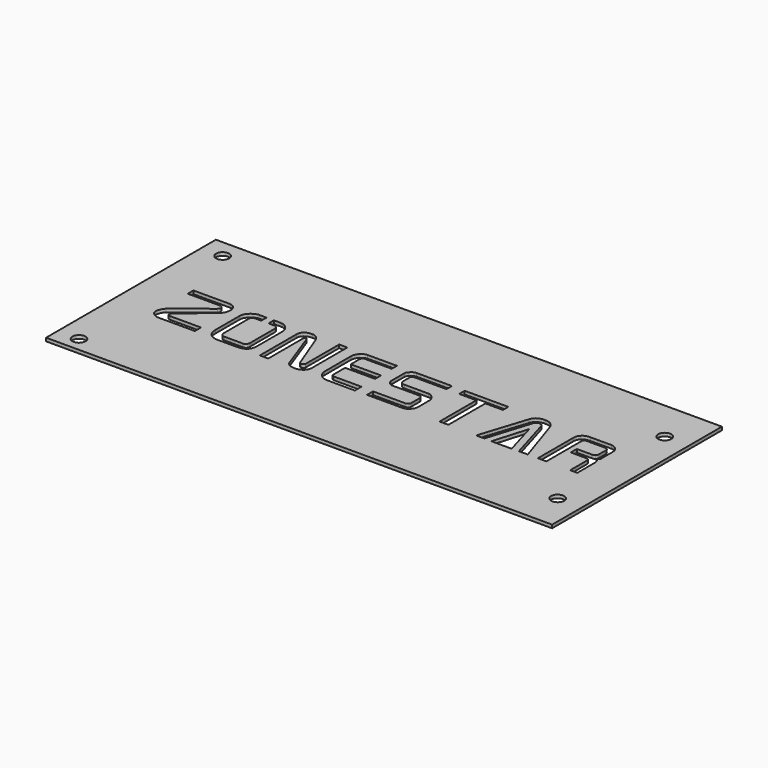
from build123d import *

# Parameters (mm, degrees)
F0_W     = 155
F0_H     = 65
F0_R     = 2
F1_DEPTH = 1


# Not quite as in the source:
# - the dataset's text gives a spline's control points without its knots; the knots are read off the source's solid


with BuildPart() as f1:
    # F0 (on Top) → F1 (new body)
    with BuildSketch(Plane.XY):
        with Locations((0.0922121108, -0.4517037495)):
            Rectangle(F0_W, F0_H)
        with Locations((-70.8632841706, -28.5362548381)):
            Circle(F0_R, mode=Mode.SUBTRACT)
        with Locations((70.1367158294, -21.5362548381)):
            Circle(F0_R, mode=Mode.SUBTRACT)
        Polygon((45.469336, -8.307439), (39.270354, -8.307439), (42.393256, 2.334635), align=None, mode=Mode.SUBTRACT)
        with BuildLine():
            add(Edge.make_bspline(
                [(-54.423643, 5.266161), (-54.520325, 5.636939), (-54.790085, 6.060127), (-55.30921, 5.999047)],
                knots=[0, 0, 0, 0, 1, 1, 1, 1], degree=3))
            Line((-55.30921, 5.999047), (-65.172596, 5.999047))
            Line((-65.172596, 5.999047), (-65.172596, 8.167165))
            Line((-65.172596, 8.167165), (-54.026665, 8.167165))
            add(Edge.make_bspline(
                [(-54.026665, 8.167165), (-52.805193, 8.228245), (-51.793658, 6.852856), (-51.797479, 5.785286)],
                knots=[0, 0, 0, 0, 1, 1, 1, 1], degree=3))
            add(Edge.make_bspline(
                [(-51.797479, 5.785286), (-51.800629, 4.896518), (-52.07231, 3.892018), (-52.74412, 3.250733)],
                knots=[0, 0, 0, 0, 1, 1, 1, 1], degree=3))
            Line((-52.74412, 3.250733), (-61.294422, -4.139179))
            add(Edge.make_bspline(
                [(-61.294422, -4.139179), (-61.2949949402, -4.1395245064), (-61.2950082917, -4.1395281699), (-61.3406298874, -4.1671100697), (-62.1897265938, -4.692143), (-62.027305, -5.207952)],
                knots=[0, 0, 0, 0, 0.0208333333, 0.03125, 1, 1, 1, 1], degree=3))
            add(Edge.make_bspline(
                [(-62.027305, -5.207952), (-61.8797565625, -5.6765360625), (-61.2435394271, -5.6963794323), (-61.1740917839, -5.6965692578), (-61.1740246232, -5.6965409216), (-61.172275, -5.69654)],
                knots=[0, 0, 0, 0, 0.9375, 0.9583333333, 1, 1, 1, 1], degree=3))
            Line((-61.172275, -5.69654), (-51.766942, -5.69654))
            Line((-51.766942, -5.69654), (-51.766942, -8.047872))
            Line((-51.766942, -8.047872), (-62.973946, -8.047872))
            add(Edge.make_bspline(
                [(-62.973946, -8.047872), (-64.042733, -8.078322), (-65.507059, -6.99161), (-65.539036, -5.940845)],
                knots=[0, 0, 0, 0, 1, 1, 1, 1], degree=3))
            add(Edge.make_bspline(
                [(-65.539036, -5.940845), (-65.565623, -5.067222), (-64.989373, -3.83381), (-64.348102, -3.284142)],
                knots=[0, 0, 0, 0, 1, 1, 1, 1], degree=3))
            Line((-64.348102, -3.284142), (-54.790085, 4.319531))
            add(Edge.make_bspline(
                [(-54.790085, 4.319531), (-54.423643, 4.624895), (-54.338273, 4.938748), (-54.423643, 5.266161)],
                knots=[0, 0, 0, 0, 1, 1, 1, 1], degree=3))
        make_face(mode=Mode.SUBTRACT)
        with BuildLine():
            Line((-38.636265, 6.060218), (-40.482756, 6.059882))
            Line((-40.482756, 6.059882), (-40.482755, 8.106095))
            Line((-40.482755, 8.106095), (-38.345683, 8.10592))
            add(Edge.make_bspline(
                [(-35.246532, 4.981721), (-35.246532, 6.428433), (-36.834187, 8.10592), (-38.345683, 8.10592)],
                knots=[0, 0, 0, 0, 1, 1, 1, 1], degree=3))
            Line((-35.246532, 4.981721), (-35.246532, -4.812387))
            add(Edge.make_bspline(
                [(-38.701388, -8.200429), (-36.69326, -8.157304), (-35.268125, -7.360324), (-35.246532, -4.812387)],
                knots=[0, 0, 0, 0, 1, 1, 1, 1], degree=3))
            Line((-38.701388, -8.200429), (-44.697956, -8.200429))
            add(Edge.make_bspline(
                [(-48.316136, -4.465362), (-48.251358, -6.879897), (-46.814048, -8.200429), (-44.697956, -8.200429)],
                knots=[0, 0, 0, 0, 1, 1, 1, 1], degree=3))
            Line((-48.316136, -4.465362), (-48.302118, 4.692146))
            add(Edge.make_bspline(
                [(-45.033966, 8.10592), (-45.984047, 8.10592), (-48.345306, 6.873016), (-48.302118, 4.692146)],
                knots=[0, 0, 0, 0, 1, 1, 1, 1], degree=3))
            Line((-45.033966, 8.10592), (-42.724205, 8.10592))
            Line((-42.724205, 8.10592), (-42.744882, 6.059882))
            Line((-42.744882, 6.059882), (-44.712989, 6.060218))
            add(Edge.make_bspline(
                [(-45.690264, 5.082949), (-45.690264, 5.464662), (-45.323727, 6.060218), (-44.712989, 6.060218)],
                knots=[0, 0, 0, 0, 1, 1, 1, 1], degree=3))
            Line((-45.690264, 5.082949), (-45.690264, -4.50575))
            add(Edge.make_bspline(
                [(-44.438112, -5.910207), (-45.270239, -5.902257), (-45.629189, -5.368415), (-45.690264, -4.50575)],
                knots=[0, 0, 0, 0, 1, 1, 1, 1], degree=3))
            Line((-44.438112, -5.910207), (-38.727779, -5.910207))
            add(Edge.make_bspline(
                [(-37.597871, -4.597264), (-37.636046, -5.467557), (-37.941457, -5.910207), (-38.727779, -5.910207)],
                knots=[0, 0, 0, 0, 1, 1, 1, 1], degree=3))
            Line((-37.597871, -4.597264), (-37.597871, 4.930313))
            add(Edge.make_bspline(
                [(-38.636265, 6.060218), (-37.949187, 6.051991), (-37.605504, 5.487612), (-37.597871, 4.930313)],
                knots=[0, 0, 0, 0, 1, 1, 1, 1], degree=3))
        make_face(mode=Mode.SUBTRACT)
        with BuildLine():
            add(Edge.make_bspline(
                [(-28.782152, 5.759499), (-29.006319, 5.729049), (-29.165424, 5.484194), (-29.170821, 5.198091)],
                knots=[0, 0, 0, 0, 1, 1, 1, 1], degree=3))
            Line((-29.170821, 5.198091), (-29.170821, -8.211027))
            Line((-29.170821, -8.211027), (-31.74036, -8.211027))
            Line((-31.74036, -8.211027), (-31.74036, 5.910654))
            add(Edge.make_bspline(
                [(-31.74036, 5.910654), (-31.675598, 7.357366), (-30.714749, 8.210275), (-28.825337, 8.264266)],
                knots=[0, 0, 0, 0, 1, 1, 1, 1], degree=3))
            add(Edge.make_bspline(
                [(-28.825337, 8.264266), (-26.9949700938, 8.31657075), (-26.2305613594, 6.1368576556), (-26.1915039655, 6.0201141621), (-26.1915066754, 6.0200826051), (-26.191019, 6.018617)],
                knots=[0, 0, 0, 0, 0.96875, 0.9791666667, 1, 1, 1, 1], degree=3))
            Line((-26.191019, 6.018617), (-21.937244, -5.036892))
            add(Edge.make_bspline(
                [(-21.937244, -5.036892), (-21.834677, -5.263602), (-21.553159, -5.453479), (-21.089727, -5.366187)],
                knots=[0, 0, 0, 0, 1, 1, 1, 1], degree=3))
            add(Edge.make_bspline(
                [(-21.089727, -5.366187), (-20.671826, -5.28752), (-20.468935, -5.047684), (-20.468935, -4.712982)],
                knots=[0, 0, 0, 0, 1, 1, 1, 1], degree=3))
            Line((-20.468935, -4.712982), (-20.468935, 8.091524))
            Line((-20.468935, 8.091524), (-17.964172, 8.091524))
            Line((-17.964172, 8.091524), (-17.964172, -5.533519))
            add(Edge.make_bspline(
                [(-17.964172, -5.533519), (-17.942573, -7.174572), (-19.608218, -8.198607), (-20.911044, -8.198607)],
                knots=[0, 0, 0, 0, 1, 1, 1, 1], degree=3))
            add(Edge.make_bspline(
                [(-20.911044, -8.198607), (-22.213871, -8.198607), (-23.402846, -7.8026), (-23.858999, -6.742715)],
                knots=[0, 0, 0, 0, 1, 1, 1, 1], degree=3))
            Line((-23.858999, -6.742715), (-28.263925, 5.327641))
            add(Edge.make_bspline(
                [(-28.263925, 5.327641), (-28.39888, 5.640739), (-28.557983, 5.790003), (-28.782152, 5.759499)],
                knots=[0, 0, 0, 0, 1, 1, 1, 1], degree=3))
        make_face(mode=Mode.SUBTRACT)
        with BuildLine():
            Line((-2.784456, 6.083385), (-11.054481, 6.083385))
            add(Edge.make_bspline(
                [(-11.702271, 5.737913), (-11.544786, 5.939612), (-11.351384, 6.083385), (-11.054481, 6.083385)],
                knots=[0, 0, 0, 0, 1, 1, 1, 1], degree=3))
            add(Edge.make_bspline(
                [(-11.896604, 4.96057), (-11.891354, 5.268261), (-11.859779, 5.536203), (-11.702271, 5.737913)],
                knots=[0, 0, 0, 0, 1, 1, 1, 1], degree=3))
            Line((-11.896604, 4.96057), (-11.896604, 1.80802))
            Line((-11.896604, 1.80802), (-2.633301, 1.80802))
            Line((-2.633301, 1.80802), (-2.633301, -0.459213))
            Line((-2.633301, -0.459213), (-11.810234, -0.459213))
            Line((-11.810234, -0.459213), (-11.810234, -4.993707))
            add(Edge.make_bspline(
                [(-11.540324, -5.506534), (-11.698656, -5.377504), (-11.815633, -5.242024), (-11.810234, -4.993707)],
                knots=[0, 0, 0, 0, 1, 1, 1, 1], degree=3))
            add(Edge.make_bspline(
                [(-10.881741, -5.663082), (-11.167851, -5.657832), (-11.381991, -5.635557), (-11.540324, -5.506534)],
                knots=[0, 0, 0, 0, 1, 1, 1, 1], degree=3))
            Line((-10.881741, -5.663082), (-2.633301, -5.663082))
            Line((-2.633301, -5.663082), (-2.633301, -8.189427))
            Line((-2.633301, -8.189427), (-11.227228, -8.189427))
            add(Edge.make_bspline(
                [(-13.451282, -7.239349), (-12.872516, -7.802097), (-11.993773, -8.162442), (-11.227228, -8.189427)],
                knots=[0, 0, 0, 0, 1, 1, 1, 1], degree=3))
            add(Edge.make_bspline(
                [(-14.466143, -5.036892), (-14.449951, -5.862807), (-14.030051, -6.676602), (-13.451282, -7.239349)],
                knots=[0, 0, 0, 0, 1, 1, 1, 1], degree=3))
            Line((-14.466143, -5.036892), (-14.466143, 5.176496))
            add(Edge.make_bspline(
                [(-13.616615, 7.184624), (-14.104807, 6.682724), (-14.468763, 5.882731), (-14.466143, 5.176496)],
                knots=[0, 0, 0, 0, 1, 1, 1, 1], degree=3))
            add(Edge.make_bspline(
                [(-11.745456, 8.091524), (-12.522793, 8.069983), (-13.128423, 7.686523), (-13.616615, 7.184624)],
                knots=[0, 0, 0, 0, 1, 1, 1, 1], degree=3))
            Line((-11.745456, 8.091524), (-2.784456, 8.091524))
            Line((-2.784456, 8.091524), (-2.784456, 6.083385))
        make_face(mode=Mode.SUBTRACT)
        with Locations((-70.8632841706, 26.4637451619)):
            Circle(F0_R, mode=Mode.SUBTRACT)
        with BuildLine():
            add(Edge.make_bspline(
                [(1.598881, 7.314182), (1.958971, 7.680189), (2.396462, 8.104167), (3.175141, 8.134707)],
                knots=[0, 0, 0, 0, 1, 1, 1, 1], degree=3))
            Line((3.175141, 8.134707), (14.036327, 8.134707))
            Line((14.036327, 8.134707), (14.036327, 6.040211))
            Line((14.036327, 6.040211), (4.125234, 6.040211))
            add(Edge.make_bspline(
                [(4.125234, 6.040211), (3.850397, 6.024941), (3.721074, 5.94307), (3.585414, 5.802682)],
                knots=[0, 0, 0, 0, 1, 1, 1, 1], degree=3))
            add(Edge.make_bspline(
                [(3.585414, 5.802682), (3.449762, 5.662334), (3.361854, 5.484259), (3.369482, 5.262861)],
                knots=[0, 0, 0, 0, 1, 1, 1, 1], degree=3))
            Line((3.369482, 5.262861), (3.369482, 2.563776))
            add(Edge.make_bspline(
                [(3.369482, 2.563776), (3.392357, 2.174428), (3.530417, 2.023619), (3.760562, 1.84596)],
                knots=[0, 0, 0, 0, 1, 1, 1, 1], degree=3))
            add(Edge.make_bspline(
                [(3.760562, 1.84596), (3.990684, 1.668301), (4.271777, 1.570501), (4.729839, 1.570501)],
                knots=[0, 0, 0, 0, 1, 1, 1, 1], degree=3))
            Line((4.729839, 1.570501), (12.092972, 1.570501))
            add(Edge.make_bspline(
                [(12.092972, 1.570501), (12.843482, 1.570501), (13.360134, 1.120618), (13.788002, 0.631214)],
                knots=[0, 0, 0, 0, 1, 1, 1, 1], degree=3))
            add(Edge.make_bspline(
                [(13.788002, 0.631214), (14.215869, 0.141821), (14.511354, -0.44272), (14.511354, -1.23656)],
                knots=[0, 0, 0, 0, 1, 1, 1, 1], degree=3))
            Line((14.511354, -1.23656), (14.511354, -5.036892))
            add(Edge.make_bspline(
                [(14.511354, -5.036892), (14.511354, -6.115047), (14.283234, -6.557255), (13.838267, -7.102385)],
                knots=[0, 0, 0, 0, 1, 1, 1, 1], degree=3))
            add(Edge.make_bspline(
                [(13.838267, -7.102385), (13.393307, -7.647522), (12.782012, -8.124657), (11.963402, -8.124657)],
                knots=[0, 0, 0, 0, 1, 1, 1, 1], degree=3))
            Line((11.963402, -8.124657), (1.037469, -8.124657))
            Line((1.037469, -8.124657), (1.037469, -5.814222))
            Line((1.037469, -5.814222), (10.862184, -5.814222))
            add(Edge.make_bspline(
                [(10.862184, -5.814222), (11.327859, -5.814222), (11.522844, -5.613829), (11.727422, -5.398722)],
                knots=[0, 0, 0, 0, 1, 1, 1, 1], degree=3))
            add(Edge.make_bspline(
                [(11.727422, -5.398722), (11.931999, -5.18363), (11.941809, -5.019957), (11.941809, -4.561842)],
                knots=[0, 0, 0, 0, 1, 1, 1, 1], degree=3))
            Line((11.941809, -4.561842), (11.941809, -1.603631))
            add(Edge.make_bspline(
                [(11.941809, -1.603631), (11.941809, -1.2472), (11.859647, -1.105843), (11.671899, -0.918077)],
                knots=[0, 0, 0, 0, 1, 1, 1, 1], degree=3))
            add(Edge.make_bspline(
                [(11.671899, -0.918077), (11.484129, -0.730289), (11.250886, -0.588775), (10.818984, -0.588775)],
                knots=[0, 0, 0, 0, 1, 1, 1, 1], degree=3))
            Line((10.818984, -0.588775), (2.829676, -0.588775))
            add(Edge.make_bspline(
                [(2.829676, -0.588775), (2.211294, -0.565937), (1.821676, -0.276933), (1.508574, 0.056398)],
                knots=[0, 0, 0, 0, 1, 1, 1, 1], degree=3))
            add(Edge.make_bspline(
                [(1.508574, 0.056398), (1.195464, 0.389723), (1.015884, 0.770604), (1.015884, 1.289787)],
                knots=[0, 0, 0, 0, 1, 1, 1, 1], degree=3))
            Line((1.015884, 1.289787), (1.015884, 6.148175))
            add(Edge.make_bspline(
                [(1.015884, 6.148175), (1.038759, 6.766545), (1.238784, 6.948176), (1.598881, 7.314182)],
                knots=[0, 0, 0, 0, 1, 1, 1, 1], degree=3))
        make_face(mode=Mode.SUBTRACT)
        Polygon((17.933274, 6.014317), (17.948559, 8.121354), (31.308407, 8.121354), (31.308407, 6.060127), (25.918651, 6.060127), (25.918651, -8.078405), (23.216154, -8.078405), (23.216154, 6.014317), align=None, mode=Mode.SUBTRACT)
        with BuildLine():
            add(Edge.make_bspline(
                [(42.387632, 8.307439), (43.664289, 8.297359), (44.948409, 7.879826), (45.604951, 6.169771)],
                knots=[0, 0, 0, 0, 1, 1, 1, 1], degree=3))
            Line((45.604951, 6.169771), (50.355369, -8.232627))
            Line((50.355369, -8.232627), (47.634669, -8.232627))
            Line((47.634669, -8.232627), (43.638699, 5.299728))
            add(Edge.make_bspline(
                [(43.638699, 5.299728), (43.402036, 5.994438), (42.900054, 6.068016), (42.470282, 6.06179)],
                knots=[0, 0, 0, 0, 1, 1, 1, 1], degree=3))
            add(Edge.make_bspline(
                [(42.470282, 6.06179), (42.040547, 6.05639), (41.523062, 5.980074), (41.263502, 5.292956)],
                knots=[0, 0, 0, 0, 1, 1, 1, 1], degree=3))
            Line((41.263502, 5.292956), (37.054202, -8.232627))
            Line((37.054202, -8.232627), (34.549449, -8.232627))
            Line((34.549449, -8.232627), (39.191904, 6.256136))
            add(Edge.make_bspline(
                [(39.191904, 6.256136), (39.703389, 7.844041), (41.110966, 8.317529), (42.387632, 8.307439)],
                knots=[0, 0, 0, 0, 1, 1, 1, 1], degree=3))
        make_face(mode=Mode.SUBTRACT)
        with BuildLine():
            Line((56.055527, -8.232612), (53.443134, -8.23667))
            Line((53.443134, -8.23667), (53.443134, 5.306053))
            add(Edge.make_bspline(
                [(53.443134, 5.306053), (53.443134, 6.367235), (53.682497, 6.778952), (54.226802, 7.306775)],
                knots=[0, 0, 0, 0, 1, 1, 1, 1], degree=3))
            add(Edge.make_bspline(
                [(54.226802, 7.306775), (54.771092, 7.834589), (55.333329, 8.082571), (56.487699, 8.082571)],
                knots=[0, 0, 0, 0, 1, 1, 1, 1], degree=3))
            Line((56.487699, 8.082571), (62.861529, 8.113111))
            add(Edge.make_bspline(
                [(62.861529, 8.113111), (63.609684, 8.113111), (64.194497, 7.772344), (64.636074, 7.319427)],
                knots=[0, 0, 0, 0, 1, 1, 1, 1], degree=3))
            add(Edge.make_bspline(
                [(64.636074, 7.319427), (65.077652, 6.866491), (65.387882, 6.31599), (65.387882, 5.543582)],
                knots=[0, 0, 0, 0, 1, 1, 1, 1], degree=3))
            Line((65.387882, 5.543582), (65.387882, 1.073873))
            add(Edge.make_bspline(
                [(65.387882, 1.073873), (65.387882, 0.844859), (65.237446, 0.660768), (65.112189, 0.53646)],
                knots=[0, 0, 0, 0, 1, 1, 1, 1], degree=3))
            add(Edge.make_bspline(
                [(65.112189, 0.53646), (64.99478775, 0.4199034375), (64.6685062161, 0.2504037995), (64.6330680026, 0.2322307188), (64.6330362965, 0.2322178923), (64.632144, 0.231761)],
                knots=[0, 0, 0, 0, 0.9375, 0.9583333333, 1, 1, 1, 1], degree=3))
            add(Edge.make_bspline(
                [(64.632144, 0.231761), (64.6333609194, 0.2307467792), (64.6334045469, 0.2307197448), (64.6817323021, 0.1903671901), (65.126441375, -0.1869175625), (65.280152, -0.469466)],
                knots=[0, 0, 0, 0, 0.0416666667, 0.0625, 1, 1, 1, 1], degree=3))
            add(Edge.make_bspline(
                [(65.280152, -0.469466), (65.444124, -0.770873), (65.539036, -1.10816), (65.539036, -1.58204)],
                knots=[0, 0, 0, 0, 1, 1, 1, 1], degree=3))
            Line((65.539036, -1.58204), (65.539036, -8.253425))
            Line((65.539036, -8.253425), (63.354219, -8.253425))
            Line((63.354219, -8.253425), (63.354219, -1.668411))
            add(Edge.make_bspline(
                [(63.354219, -1.668411), (63.354219, -1.416037), (63.261091, -1.295952), (63.128026, -1.161526)],
                knots=[0, 0, 0, 0, 1, 1, 1, 1], degree=3))
            add(Edge.make_bspline(
                [(63.128026, -1.161526), (62.994984, -1.027099), (62.844189, -0.977434), (62.576866, -0.977434)],
                knots=[0, 0, 0, 0, 1, 1, 1, 1], degree=3))
            Line((62.576866, -0.977434), (57.718209, -0.977434))
            Line((57.718209, -0.977434), (57.710259, 1.332979))
            Line((57.710259, 1.332979), (62.446996, 1.332979))
            add(Edge.make_bspline(
                [(62.446996, 1.332979), (62.839021, 1.332979), (63.042849, 1.436234), (63.257491, 1.636598)],
                knots=[0, 0, 0, 0, 1, 1, 1, 1], degree=3))
            add(Edge.make_bspline(
                [(63.257491, 1.636598), (63.472111, 1.836952), (63.591414, 2.138162), (63.591414, 2.498988)],
                knots=[0, 0, 0, 0, 1, 1, 1, 1], degree=3))
            Line((63.591414, 2.498988), (63.591414, 5.068533))
            add(Edge.make_bspline(
                [(63.591414, 5.068533), (63.591414, 5.443856), (63.465639, 5.672251), (63.247231, 5.848719)],
                knots=[0, 0, 0, 0, 1, 1, 1, 1], degree=3))
            add(Edge.make_bspline(
                [(63.247231, 5.848719), (63.028824, 6.025187), (62.820519, 6.040212), (62.339034, 6.040212)],
                knots=[0, 0, 0, 0, 1, 1, 1, 1], degree=3))
            Line((62.339034, 6.040212), (56.962426, 6.040212))
            add(Edge.make_bspline(
                [(56.962426, 6.040212), (56.587104, 6.040212), (56.370174, 5.877023), (56.223264, 5.653073)],
                knots=[0, 0, 0, 0, 1, 1, 1, 1], degree=3))
            add(Edge.make_bspline(
                [(56.223264, 5.653073), (56.076339, 5.429131), (56.055527, 5.212144), (56.055527, 4.852609)],
                knots=[0, 0, 0, 0, 1, 1, 1, 1], degree=3))
            Line((56.055527, 4.852609), (56.055527, -8.232612))
        make_face(mode=Mode.SUBTRACT)
        with Locations((70.1367158294, 19.4637451619)):
            Circle(F0_R, mode=Mode.SUBTRACT)
    extrude(amount=F1_DEPTH)


solid = f1.part
